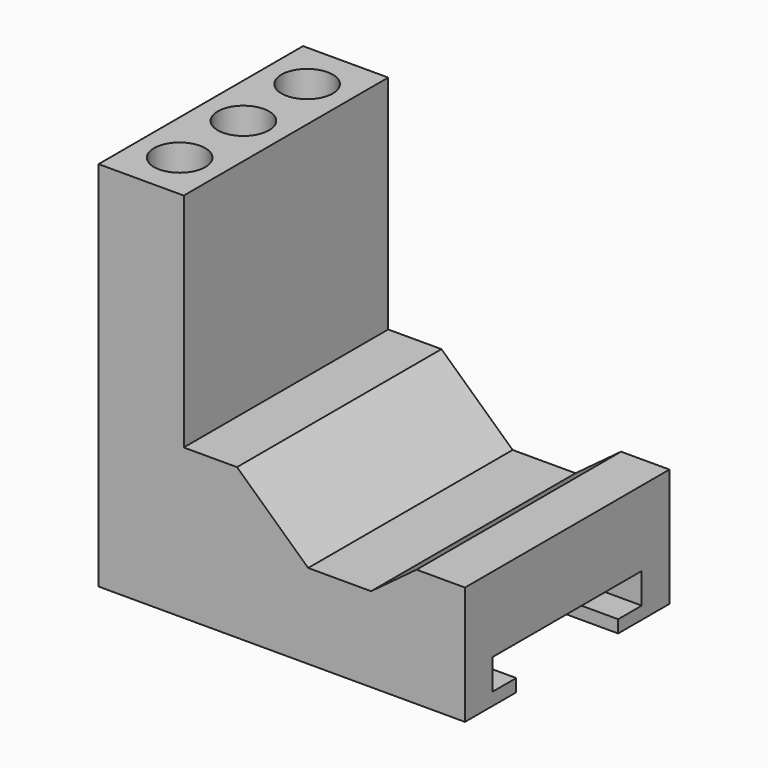
from build123d import *

# Parameters (mm, degrees)
F1_DEPTH = 26.4
F2_R     = 2.65
F3_DEPTH = 32.25
F4_DEPTH = 40
F5_W     = 20
F5_H     = 13.16
F6_DEPTH = 4.45
F7_W     = 3.045
F7_H     = 3.15
F8_DEPTH = 20


# Not quite as in the source:
# - a feature names something its author has since deleted; it is built from what else it names


with BuildPart() as f1:
    # F0 (on Front) → F1 (new body)
    with BuildSketch(Plane.XZ):
        Polygon((-12.7175080026, 22.9085270187), (-21.5175080026, 22.9085270187), (-21.5175080026, -15.5114729813), (16.3324919974, -15.5114729813), (16.3324919974, -3.2914729813), (11.3324919974, -3.2914729813), (6.6349683525, -6.7779857958), (0.1349683525, -6.7779857958), (-7.2175080026, 0), (-12.7175080026, 0), align=None)
    extrude(amount=F1_DEPTH)

    # F2 (on face) → F3 (cut)
    with BuildSketch(Plane.XY.offset(22.9085270187)):
        with Locations((-17.1175080026, -4.97)):
            Circle(F2_R)
        with Locations((-17.1175080026, -21.43)):
            Circle(F2_R)
    extrude(amount=-F3_DEPTH, mode=Mode.SUBTRACT)

    # F2 (on face) → F4 (cut)
    with BuildSketch(Plane.XY.offset(22.9085270187)):
        with Locations((-17.1175080026, -13.2)):
            Circle(F2_R)
    extrude(amount=-F4_DEPTH, mode=Mode.SUBTRACT)

    # F5 (on face) → F6 (cut)
    with BuildSketch(Plane(origin=(0, 0, -15.5114729813), x_dir=(1, 0, 0), z_dir=(0, 0, -1))):
        with Locations((6.3324919974, 13.2)):
            Rectangle(F5_W, F5_H)
    extrude(amount=-F6_DEPTH, mode=Mode.SUBTRACT)

    # F7 (on face) → F8 (cut)
    with BuildSketch(Plane.YZ.offset(16.3324919974)):
        with Locations((-5.0975, -12.6364729813)):
            Rectangle(F7_W, F7_H)
        with Locations((-21.3025, -12.6364729813)):
            Rectangle(F7_W, F7_H)
    extrude(amount=-F8_DEPTH, mode=Mode.SUBTRACT)


solid = f1.part
